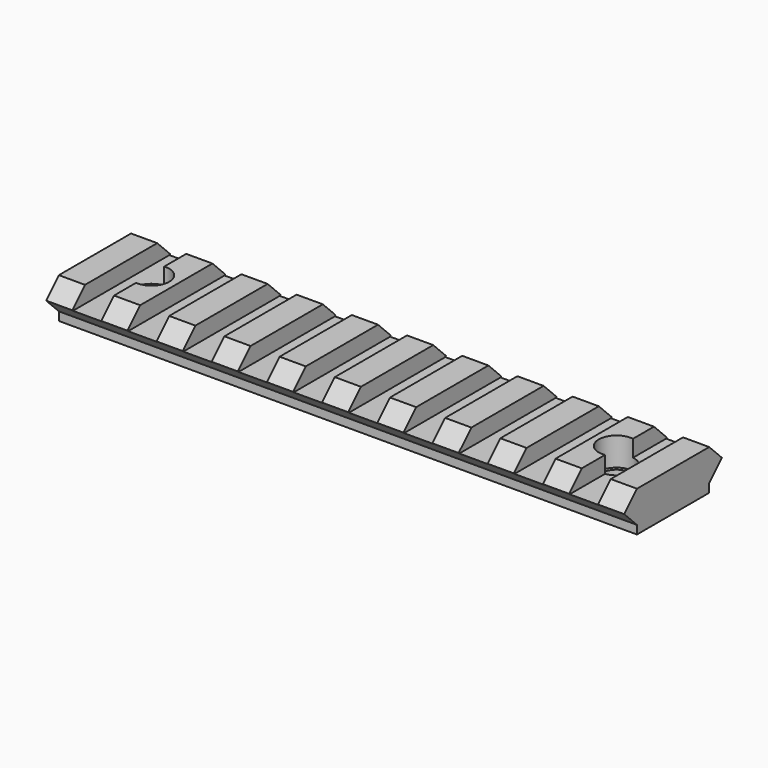
from build123d import *

# Parameters (mm, degrees)
F1_DEPTH = 103.759
F2_W     = 5.207
F2_H     = 2.8575
F2_H_2   = 16.2052
F2_H_3   = 2.9408035447
F3_DEPTH = 2.9972
F4_R     = 2.54
F5_DEPTH = 7.239
F6_R     = 3.175
F7_DEPTH = 5.08


with BuildPart() as f1:
    # F0 (on Right) → F1 (new body)
    with BuildSketch(Plane.YZ):
        Polygon((0, 1.524), (0, 0), (16.2052, 0), (16.2052, 1.524), (19.0627, 4.3815), (16.2052, 7.239), (0, 7.239), (-2.8575, 4.3815), align=None)
    extrude(amount=F1_DEPTH)

    # F2 (on face) → F3 (cut)
    with BuildSketch(Plane.XY.offset(7.239)):
        with Locations((7.3025, -1.42875)):
            Rectangle(F2_W, F2_H)
        Polygon((4.699, 16.2052), (4.699, 8.1026), (4.699, 0), (9.906, 0), (9.906, 16.2052), align=None)
        with Locations((7.3025, 17.63395)):
            Rectangle(F2_W, F2_H)
        with Locations((17.2085, 17.63395)):
            Rectangle(F2_W, F2_H)
        with Locations((17.2085, 8.1026)):
            Rectangle(F2_W, F2_H_2)
        with Locations((17.2085, -1.42875)):
            Rectangle(F2_W, F2_H)
        with Locations((27.1145, 17.63395)):
            Rectangle(F2_W, F2_H)
        with Locations((27.1145, 8.1026)):
            Rectangle(F2_W, F2_H_2)
        with Locations((27.1145, -1.42875)):
            Rectangle(F2_W, F2_H)
        with Locations((37.0205, 17.63395)):
            Rectangle(F2_W, F2_H)
        with Locations((37.0205, 8.1026)):
            Rectangle(F2_W, F2_H_2)
        with Locations((37.0205, -1.42875)):
            Rectangle(F2_W, F2_H)
        with Locations((46.9265, 17.63395)):
            Rectangle(F2_W, F2_H)
        with Locations((46.9265, 8.1026)):
            Rectangle(F2_W, F2_H_2)
        with Locations((46.9265, -1.42875)):
            Rectangle(F2_W, F2_H)
        with Locations((56.8325, 17.63395)):
            Rectangle(F2_W, F2_H)
        with Locations((56.8325, 8.1026)):
            Rectangle(F2_W, F2_H_2)
        with Locations((56.8325, -1.42875)):
            Rectangle(F2_W, F2_H)
        with Locations((66.7385, 17.63395)):
            Rectangle(F2_W, F2_H)
        with Locations((66.7385, 8.1026)):
            Rectangle(F2_W, F2_H_2)
        with Locations((66.7385, -1.42875)):
            Rectangle(F2_W, F2_H)
        with Locations((76.6445, 17.63395)):
            Rectangle(F2_W, F2_H)
        with Locations((76.6445, 8.1026)):
            Rectangle(F2_W, F2_H_2)
        with Locations((76.6445, -1.42875)):
            Rectangle(F2_W, F2_H)
        with Locations((86.5505, -1.42875)):
            Rectangle(F2_W, F2_H)
        with Locations((86.5505, 8.1026)):
            Rectangle(F2_W, F2_H_2)
        with Locations((86.5505, 17.63395)):
            Rectangle(F2_W, F2_H)
        with Locations((96.4565, 17.6756017723)):
            Rectangle(F2_W, F2_H_3)
        with Locations((96.4565, 8.1026)):
            Rectangle(F2_W, F2_H_2)
        with Locations((96.4565, -1.4704017723)):
            Rectangle(F2_W, F2_H_3)
    extrude(amount=-F3_DEPTH, mode=Mode.SUBTRACT)

    # F4 (on face) → F5 (cut)
    with BuildSketch(Plane(origin=(0, 0, 0), x_dir=(1, 0, 0), z_dir=(0, 0, -1))):
        with Locations((93.4012121817, -8.3558605984)):
            Circle(F4_R)
        with Locations((10.16, -8.1026)):
            Circle(F4_R)
    extrude(amount=-F5_DEPTH, mode=Mode.SUBTRACT)

    # F6 (on face) → F7 (cut)
    with BuildSketch(Plane.XY.offset(7.239)):
        with Locations((93.4012121817, 8.3558605984)):
            Circle(F6_R)
        with Locations((10.16, 8.1026)):
            Circle(F6_R)
    extrude(amount=-F7_DEPTH, mode=Mode.SUBTRACT)


with BuildPart() as f8_1:
    # F8: copy of F1
    add(f1.part)


solid = Compound([f1.part, f8_1.part])
